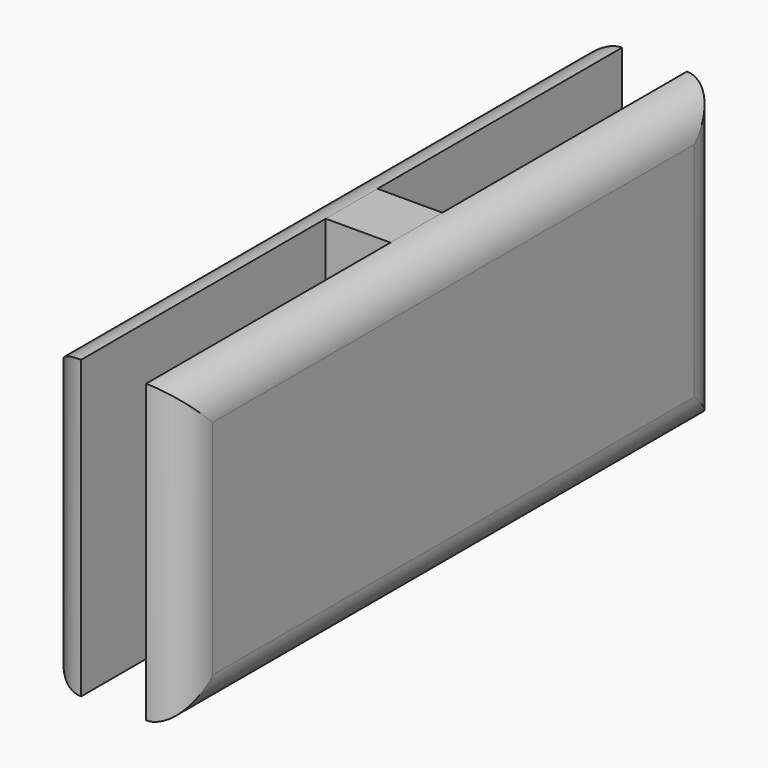
from build123d import *

# Parameters (mm, degrees)
F1_DEPTH = 8
F2_R     = 0.99999


# Not quite as in the source:
# - a fillet or chamfer is up to 0.001 mm smaller than in the source, because OpenCascade refuses the exact size


with BuildPart() as f1:
    # F0 (on Top) → F1 (new body)
    with BuildSketch(Plane.XY):
        Polygon((20.5548869669, -26.5982374549), (20.5548869669, -18.3482374549), (22.3048869669, -18.3482374549), (22.3048869669, -26.5982374549), (23.3048869669, -26.5982374549), (23.3048869669, -18.3482374549), (23.3048869669, -8.3482374549), (22.3048869669, -8.3482374549), (22.3048869669, -16.5982374549), (20.5548869669, -16.5982374549), (20.5548869669, -8.3482374549), (19.5548869669, -8.3482374549), (19.5548869669, -18.3482374549), (19.5548869669, -26.5982374549), align=None)
    extrude(amount=F1_DEPTH)

    # F2 (radius 1 in the source; OpenCascade refuses exactly that, so slightly less here)
    f2_edges = [f1.edges().sort_by_distance(p)[0] for p in [
        (23.304887, -26.598237, 4),
        (23.304887, -17.473237, 8),
        (23.304887, -8.348237, 4),
        (23.304887, -17.473237, 0),
        (19.554887, -26.598237, 4),
        (19.554887, -17.473237, 8),
        (19.554887, -8.348237, 4),
        (19.554887, -17.473237, 0),
    ]]
    fillet(f2_edges, radius=F2_R)


solid = f1.part
